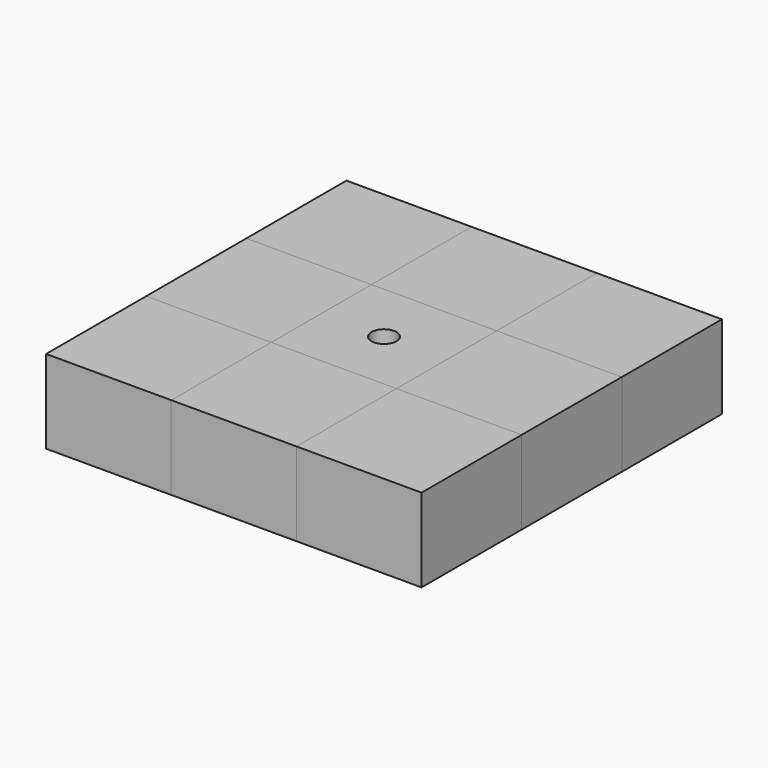
from build123d import *

# Parameters (mm, degrees)
F0_W     = 38.1
F0_H     = 38.1
F6_DEPTH = 25.4
F3_W     = 38.1
F3_H     = 38.1
F7_DEPTH = 25.4
F2_W     = 38.1
F2_H     = 38.1
F1_W     = 38.1
F1_H     = 38.1
F4_W     = 38.1
F4_H     = 38.1
F5_W     = 38.1
F5_H     = 38.1
F8_R     = 3.8061602771
F9_DEPTH = 59.436


with BuildPart() as f6:
    # F0 (on Top) → F6 (new body)
    with BuildSketch(Plane.XY):
        with Locations((0, 38.1)):
            Rectangle(F0_W, F0_H)
    extrude(amount=F6_DEPTH)


with BuildPart() as f6b:
    # F0 (on Top) → F6, piece 2 (new body)
    with BuildSketch(Plane.XY):
        with Locations((38.1, 0)):
            Rectangle(F0_W, F0_H)
    extrude(amount=F6_DEPTH)


with BuildPart() as f6c:
    # F0 (on Top) → F6, piece 3 (new body)
    with BuildSketch(Plane.XY):
        with Locations((0, -38.1)):
            Rectangle(F0_W, F0_H)
    extrude(amount=F6_DEPTH)


with BuildPart() as f6d:
    # F0 (on Top) → F6, piece 4 (new body)
    with BuildSketch(Plane.XY):
        with Locations((-38.1, 0)):
            Rectangle(F0_W, F0_H)
    extrude(amount=F6_DEPTH)


with BuildPart() as f7:
    # F3 (on face) → F7 (new body)
    with BuildSketch(Plane.XY):
        Rectangle(F3_W, F3_H)
    extrude(amount=F7_DEPTH)

    # F8 (on Top) → F9 (cut)
    with BuildSketch(Plane.XY):
        Circle(F8_R)
    extrude(amount=F9_DEPTH, mode=Mode.SUBTRACT)


with BuildPart() as f7b:
    # F2 (on face) → F7, piece 2 (new body)
    with BuildSketch(Plane.XY):
        with Locations((-38.1, 38.1)):
            Rectangle(F2_W, F2_H)
    extrude(amount=F7_DEPTH)


with BuildPart() as f7c:
    # F1 (on face) → F7, piece 3 (new body)
    with BuildSketch(Plane.XY):
        with Locations((38.1, 38.1)):
            Rectangle(F1_W, F1_H)
    extrude(amount=F7_DEPTH)


with BuildPart() as f7d:
    # F4 (on face) → F7, piece 4 (new body)
    with BuildSketch(Plane.XY):
        with Locations((38.1, -38.1)):
            Rectangle(F4_W, F4_H)
    extrude(amount=F7_DEPTH)


with BuildPart() as f7e:
    # F5 (on face) → F7, piece 5 (new body)
    with BuildSketch(Plane.XY):
        with Locations((-38.1, -38.1)):
            Rectangle(F5_W, F5_H)
    extrude(amount=F7_DEPTH)


solid = Compound([f6.part, f6b.part, f6c.part, f6d.part, f7.part, f7b.part, f7c.part, f7d.part, f7e.part])
